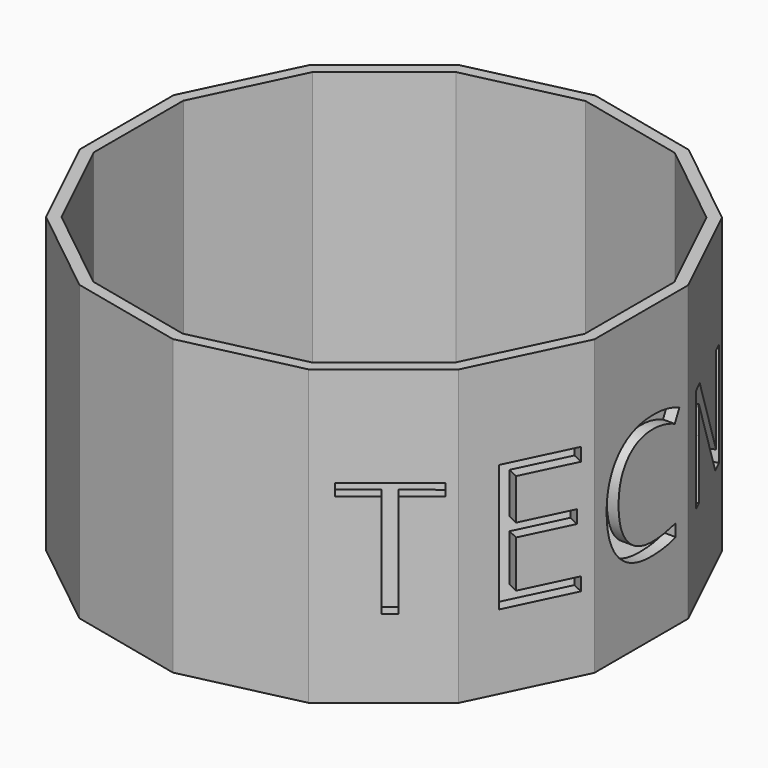
from build123d import *

# Parameters (mm, degrees)
F4_T          = -2
F5_TEXT_SIZE  = 30.3578369009
F6_DEPTH      = 25
F7_TEXT_SIZE  = 28.7319210151
F8_DEPTH      = 25
F9_TEXT_SIZE  = 24.8829433177
F10_DEPTH     = 25
F11_TEXT_SIZE = 24.1104409926
F12_DEPTH     = 25
F13_TEXT_SIZE = 27.4445007866
F14_DEPTH     = 25


# Not quite as in the source:
# - Text() gives the source's letters only with a copy of the font that has no kerning and outlines rounded to 1/6400 em; it was checked with that copy


with BuildPart() as f3:
    # F0 (on Top) → F3 section 0
    with BuildSketch(Plane.XY):
        Polygon((-19.4985582436, -40.4891733952), (0, -44.9395920743), (19.4985582436, -40.4891733952), (35.135187893, -28.019377358), (43.8128626753, -10), (43.8128626753, 10), (35.135187893, 28.019377358), (19.4985582436, 40.4891733952), (0, 44.9395920743), (-19.4985582436, 40.4891733952), (-35.135187893, 28.019377358), (-43.8128626753, 10), (-43.8128626753, -10), (-35.135187893, -28.019377358), align=None)
    # F2 (on offset) → F3 section 1
    with BuildSketch(Plane.XY.offset(50)):
        Polygon((19.4985582436, 40.4891733952), (0, 44.9395920743), (-19.4985582436, 40.4891733952), (-35.135187893, 28.019377358), (-43.8128626753, 10), (-43.8128626753, -10), (-35.135187893, -28.019377358), (-19.4985582436, -40.4891733952), (0, -44.9395920743), (19.4985582436, -40.4891733952), (35.135187893, -28.019377358), (43.8128626753, -10), (43.8128626753, 10), (35.135187893, 28.019377358), align=None)
    loft()

    # F4
    f4_openings = [f3.faces().sort_by_distance(p)[0] for p in [
        (0, 0, 50),
    ]]
    offset(amount=F4_T, openings=f4_openings)

    # F5 (on face) → F6 (cut)
    with BuildSketch(Plane(origin=(39.4740252842, -19.009688679, 0), x_dir=(0.4338837391, 0.9009688679, 0), z_dir=(0.9009688679, -0.4338837391, 0))):
        with Locations((-7.0288491366, 12.6702478155)):
            Text('E', F5_TEXT_SIZE, font='Open Sans', text_align=(TextAlign.LEFT, TextAlign.BOTTOM))
    extrude(amount=-F6_DEPTH, mode=Mode.SUBTRACT)

    # F7 (on face) → F8 (cut)
    with BuildSketch(Plane.YZ.offset(43.8128626753)):
        with Locations((-9.133663651, 12.8001691774)):
            Text('C', F7_TEXT_SIZE, font='Open Sans', text_align=(TextAlign.LEFT, TextAlign.BOTTOM))
    extrude(amount=-F8_DEPTH, mode=Mode.SUBTRACT)

    # F9 (on face) → F10 (cut)
    with BuildSketch(Plane(origin=(39.4740252842, 19.009688679, 0), x_dir=(-0.4338837391, 0.9009688679, 0), z_dir=(0.9009688679, 0.4338837391, 0))):
        with Locations((-7.9312710283, 14.0653764829)):
            Text('N', F9_TEXT_SIZE, font='Open Sans', text_align=(TextAlign.LEFT, TextAlign.BOTTOM))
    extrude(amount=-F10_DEPTH, mode=Mode.SUBTRACT)

    # F11 (on face) → F12 (cut)
    with BuildSketch(Plane(origin=(27.3168730683, 34.2542753766, 0), x_dir=(-0.7818314825, 0.6234898019, 0), z_dir=(0.6234898019, 0.7818314825, 0))):
        with Locations((-8.8701873332, 14.3130160868)):
            Text('O', F11_TEXT_SIZE, font='Open Sans', text_align=(TextAlign.LEFT, TextAlign.BOTTOM))
    extrude(amount=-F12_DEPTH, mode=Mode.SUBTRACT)

    # F13 (on face) → F14 (cut)
    with BuildSketch(Plane(origin=(27.3168730683, -34.2542753766, 0), x_dir=(0.7818314825, 0.6234898019, 0), z_dir=(0.6234898019, -0.7818314825, 0))):
        with Locations((-6.7068398538, 13.34858872)):
            Text('T', F13_TEXT_SIZE, font='Open Sans', text_align=(TextAlign.LEFT, TextAlign.BOTTOM))
    extrude(amount=-F14_DEPTH, mode=Mode.SUBTRACT)


solid = f3.part
